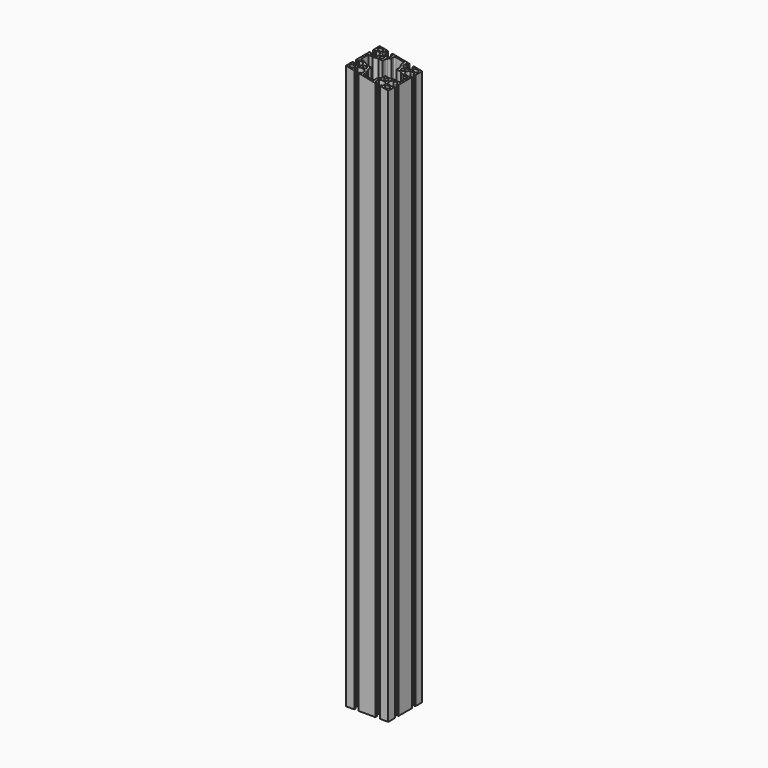
from build123d import *

# Parameters (mm, degrees)
F0_R          = 3
F0_R_2        = 2.5
F1_DEPTH      = 800
F2_R          = 2
F3_R          = 7
F6_DEPTH      = 30
F6_DEPTH_BACK = 30


# Not quite as in the source:
# - a feature names something its author has since deleted; it is built from what else it names


with BuildPart() as f1:
    # F0 (on Top) → F1 (new body)
    with BuildSketch(Plane.XY):
        with BuildLine():
            Line((18.15, -30), (30, -30))
            Line((30, -30), (30, -18.15))
            Line((30, -18.15), (27.5, -18.15))
            Line((27.5, -18.15), (27.5, -20.15))
            Line((27.5, -20.15), (21.5477069044, -20.15))
            ThreePointArc((21.5477069044, -20.15), (19.5, -15), (21.5477069044, -9.85))
            Line((21.5477069044, -9.85), (27.5, -9.85))
            Line((27.5, -9.85), (27.5, -11.85))
            Line((27.5, -11.85), (30, -11.85))
            Line((30, -11.85), (30, 11.85))
            Line((30, 11.85), (27.5, 11.85))
            Line((27.5, 11.85), (27.5, 9.85))
            Line((27.5, 9.85), (21.5477069044, 9.85))
            ThreePointArc((21.5477069044, 9.85), (19.5, 15), (21.5477069044, 20.15))
            Line((21.5477069044, 20.15), (27.5, 20.15))
            Line((27.5, 20.15), (27.5, 18.15))
            Line((27.5, 18.15), (30, 18.15))
            Line((30, 18.15), (30, 30))
            Line((30, 30), (18.15, 30))
            Line((18.15, 30), (18.15, 27.5))
            Line((18.15, 27.5), (20.15, 27.5))
            Line((20.15, 27.5), (20.15, 21.5477069044))
            ThreePointArc((20.15, 21.5477069044), (15, 19.5), (9.85, 21.5477069044))
            Line((9.85, 21.5477069044), (9.85, 27.5))
            Line((9.85, 27.5), (11.85, 27.5))
            Line((11.85, 27.5), (11.85, 30))
            Line((11.85, 30), (-11.85, 30))
            Line((-11.85, 30), (-11.85, 27.5))
            Line((-11.85, 27.5), (-9.85, 27.5))
            Line((-9.85, 27.5), (-9.85, 21.5477069044))
            ThreePointArc((-9.85, 21.5477069044), (-15, 19.5), (-20.15, 21.5477069044))
            Line((-20.15, 21.5477069044), (-20.15, 27.5))
            Line((-20.15, 27.5), (-18.15, 27.5))
            Line((-18.15, 27.5), (-18.15, 30))
            Line((-18.15, 30), (-30, 30))
            Line((-30, 30), (-30, 18.15))
            Line((-30, 18.15), (-27.5, 18.15))
            Line((-27.5, 18.15), (-27.5, 20.15))
            Line((-27.5, 20.15), (-21.5477069044, 20.15))
            ThreePointArc((-21.5477069044, 20.15), (-19.5, 15), (-21.5477069044, 9.85))
            Line((-21.5477069044, 9.85), (-27.5, 9.85))
            Line((-27.5, 9.85), (-27.5, 11.85))
            Line((-27.5, 11.85), (-30, 11.85))
            Line((-30, 11.85), (-30, -11.85))
            Line((-30, -11.85), (-27.5, -11.85))
            Line((-27.5, -11.85), (-27.5, -9.85))
            Line((-27.5, -9.85), (-21.5477069044, -9.85))
            ThreePointArc((-21.5477069044, -9.85), (-19.5, -15), (-21.5477069044, -20.15))
            Line((-21.5477069044, -20.15), (-27.5, -20.15))
            Line((-27.5, -20.15), (-27.5, -18.15))
            Line((-27.5, -18.15), (-30, -18.15))
            Line((-30, -18.15), (-30, -30))
            Line((-30, -30), (-18.15, -30))
            Line((-18.15, -30), (-18.15, -27.5))
            Line((-18.15, -27.5), (-20.15, -27.5))
            Line((-20.15, -27.5), (-20.15, -21.5477069044))
            ThreePointArc((-20.15, -21.5477069044), (-15, -19.5), (-9.85, -21.5477069044))
            Line((-9.85, -21.5477069044), (-9.85, -27.5))
            Line((-9.85, -27.5), (-11.85, -27.5))
            Line((-11.85, -27.5), (-11.85, -30))
            Line((-11.85, -30), (11.85, -30))
            Line((11.85, -30), (11.85, -27.5))
            Line((11.85, -27.5), (9.85, -27.5))
            Line((9.85, -27.5), (9.85, -21.5477069044))
            ThreePointArc((9.85, -21.5477069044), (15, -19.5), (20.15, -21.5477069044))
            Line((20.15, -21.5477069044), (20.15, -27.5))
            Line((20.15, -27.5), (18.15, -27.5))
            Line((18.15, -27.5), (18.15, -30))
        make_face()
        with Locations((-25, -25)):
            Circle(F0_R, mode=Mode.SUBTRACT)
        with Locations((-15, -15)):
            Circle(F0_R_2, mode=Mode.SUBTRACT)
        with Locations((25, -25)):
            Circle(F0_R, mode=Mode.SUBTRACT)
        with Locations((15, -15)):
            Circle(F0_R_2, mode=Mode.SUBTRACT)
        with Locations((-25, 25)):
            Circle(F0_R, mode=Mode.SUBTRACT)
        with Locations((-15, 15)):
            Circle(F0_R_2, mode=Mode.SUBTRACT)
        Polygon((-7, 22), (-7, 27.5), (0, 27.5), (7, 27.5), (7, 22), (10, 16), (10, 10), (16, 10), (22, 7), (27.5, 7), (27.5, 0), (27.5, -7), (22, -7), (16, -10), (10, -10), (10, -16), (7, -22), (7, -27.5), (0, -27.5), (-7, -27.5), (-7, -22), (-10, -16), (-10, -10), (-16, -10), (-22, -7), (-27.5, -7), (-27.5, 0), (-27.5, 7), (-22, 7), (-16, 10), (-10, 10), (-10, 16), align=None, mode=Mode.SUBTRACT)
        with Locations((15, 15)):
            Circle(F0_R_2, mode=Mode.SUBTRACT)
        with Locations((25, 25)):
            Circle(F0_R, mode=Mode.SUBTRACT)
    extrude(amount=F1_DEPTH)

    # F2
    f2_edges = [f1.edges().sort_by_distance(p)[0] for p in [
        (-7, 27.5, 400),
        (7, 27.5, 400),
    ]]
    fillet(f2_edges, radius=F2_R)

    # F3
    f3_edges = [f1.edges().sort_by_distance(p)[0] for p in [
        (-10, 16, 400),
        (10, 16, 400),
    ]]
    fillet(f3_edges, radius=F3_R)

    # F5 (on Front) → F6 (cut, two sides)
    with BuildSketch(Plane.XZ) as f6_sk:
        Polygon((92.6955789172, 775.5943319306), (113.9419287111, 882.406945313), (-8.7536502061, 906.8126133825), (-30, 800), align=None)
    extrude(amount=F6_DEPTH, mode=Mode.SUBTRACT)
    extrude(f6_sk.sketch, amount=-F6_DEPTH_BACK, mode=Mode.SUBTRACT)


solid = f1.part
